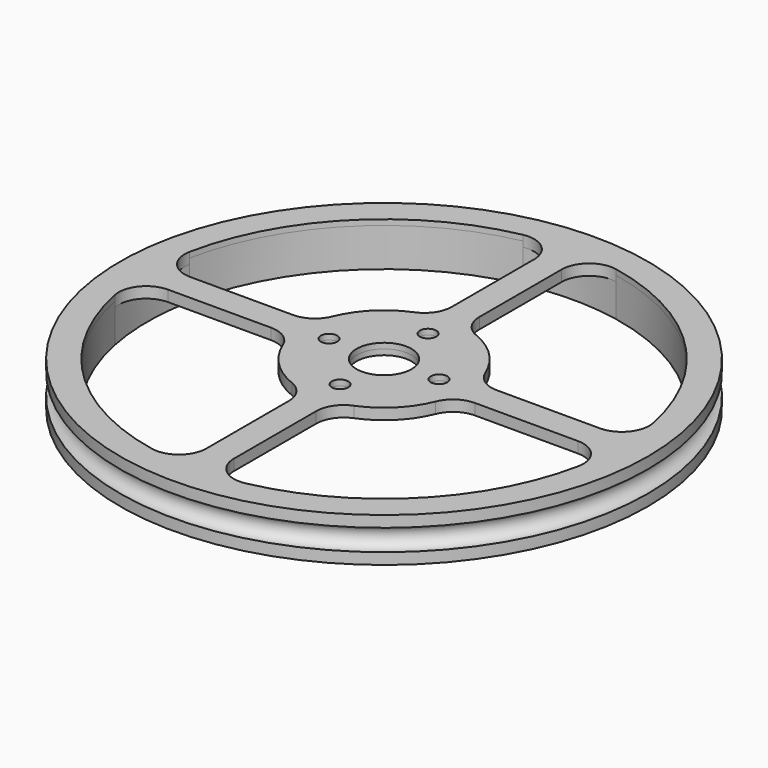
from build123d import *

# Parameters (mm, degrees)
F0_R          = 48
F1_DEPTH      = 1
F1_DEPTH_BACK = 7
F0_R_2        = 1.5
F0_R_3        = 5
F2_DEPTH      = 1
F3_DEPTH      = 1


with BuildPart() as f1:
    # F0 (on Top) → F1 (new body, two sides)
    with BuildSketch(Plane.XY) as f1_sk:
        Circle(F0_R)
        with BuildLine():
            ThreePointArc((8.4868421053, -42.1541636269), (4.2644439289, -42.7880183927), (0, -43))
            ThreePointArc((0, -43), (-4.2644439289, -42.7880183927), (-8.4868421053, -42.1541636269))
            ThreePointArc((-8.4868421053, -42.1541636269), (-30.405591591, -30.405591591), (-42.1541636269, -8.4868421053))
            ThreePointArc((-42.1541636269, -8.4868421053), (-43, 0), (-42.1541636269, 8.4868421053))
            ThreePointArc((-42.1541636269, 8.4868421053), (-30.405591591, 30.405591591), (-8.4868421053, 42.1541636269))
            ThreePointArc((-8.4868421053, 42.1541636269), (0, 43), (8.4868421053, 42.1541636269))
            ThreePointArc((8.4868421053, 42.1541636269), (30.405591591, 30.405591591), (42.1541636269, 8.4868421053))
            ThreePointArc((42.1541636269, 8.4868421053), (42.7880183927, 4.2644439289), (43, 0))
            ThreePointArc((43, 0), (42.7880183927, -4.2644439289), (42.1541636269, -8.4868421053))
            ThreePointArc((42.1541636269, -8.4868421053), (30.405591591, -30.405591591), (8.4868421053, -42.1541636269))
        make_face(mode=Mode.SUBTRACT)
    extrude(amount=F1_DEPTH)
    extrude(f1_sk.sketch, amount=-F1_DEPTH_BACK)



with BuildPart() as f2:
    # F0 (on Top) → F2 (new body, symmetric)
    with BuildSketch(Plane.XY):
        with BuildLine():
            ThreePointArc((0, -15), (2.8652589369, -14.7238001625), (5.625, -13.9053721633))
            ThreePointArc((5.625, -13.9053721633), (10.6066017178, -10.6066017178), (13.9053721633, -5.625))
            ThreePointArc((13.9053721633, -5.625), (14.7238001625, -2.8652589369), (15, 0))
            ThreePointArc((15, 0), (14.7238001625, 2.8652589369), (13.9053721633, 5.625))
            ThreePointArc((13.9053721633, 5.625), (10.6066017178, 10.6066017178), (5.625, 13.9053721633))
            ThreePointArc((5.625, 13.9053721633), (0, 15), (-5.625, 13.9053721633))
            ThreePointArc((-5.625, 13.9053721633), (-10.6066017178, 10.6066017178), (-13.9053721633, 5.625))
            ThreePointArc((-13.9053721633, 5.625), (-15, 0), (-13.9053721633, -5.625))
            ThreePointArc((-13.9053721633, -5.625), (-10.6066017178, -10.6066017178), (-5.625, -13.9053721633))
            ThreePointArc((-5.625, -13.9053721633), (-2.8652589369, -14.7238001625), (0, -15))
        make_face()
        with Locations((0, -10)):
            Circle(F0_R_2, mode=Mode.SUBTRACT)
        with Locations((-10, 0)):
            Circle(F0_R_2, mode=Mode.SUBTRACT)
        Circle(F0_R_3, mode=Mode.SUBTRACT)
        with Locations((10, 0)):
            Circle(F0_R_2, mode=Mode.SUBTRACT)
        with Locations((0, 10)):
            Circle(F0_R_2, mode=Mode.SUBTRACT)
    extrude(amount=F2_DEPTH, both=True)


with BuildPart() as f1_1:
    add(f1.part)

    add(f2.part)  # F3 merges F2
    # F0 (on Top) → F3 (join, symmetric)
    with BuildSketch(Plane.XY):
        with BuildLine():
            Line((0, -43), (0, -15))
            ThreePointArc((0, -15), (-2.8652589369, -14.7238001625), (-5.625, -13.9053721633))
            ThreePointArc((-5.625, -13.9053721633), (-3.3542190121, -15.7454112459), (-2.5, -18.5404962177))
            Line((-2.5, -18.5404962177), (-2.5, -37.2525166935))
            ThreePointArc((-2.5, -37.2525166935), (-4.3325254955, -41.1212510167), (-8.4868421053, -42.1541636269))
            ThreePointArc((-8.4868421053, -42.1541636269), (-4.2644439289, -42.7880183927), (0, -43))
        make_face()
        with BuildLine():
            ThreePointArc((2.5, -18.5404962177), (3.3542190121, -15.7454112459), (5.625, -13.9053721633))
            ThreePointArc((5.625, -13.9053721633), (2.8652589369, -14.7238001625), (0, -15))
            Line((0, -15), (0, -43))
            ThreePointArc((0, -43), (4.2644439289, -42.7880183927), (8.4868421053, -42.1541636269))
            ThreePointArc((8.4868421053, -42.1541636269), (4.3325254955, -41.1212510167), (2.5, -37.2525166935))
            Line((2.5, -37.2525166935), (2.5, -18.5404962177))
        make_face()
        with BuildLine():
            ThreePointArc((15, 0), (14.7238001625, -2.8652589369), (13.9053721633, -5.625))
            ThreePointArc((13.9053721633, -5.625), (15.7454112459, -3.3542190121), (18.5404962177, -2.5))
            Line((18.5404962177, -2.5), (37.2525166935, -2.5))
            ThreePointArc((37.2525166935, -2.5), (41.1212510167, -4.3325254955), (42.1541636269, -8.4868421053))
            ThreePointArc((42.1541636269, -8.4868421053), (42.7880183927, -4.2644439289), (43, 0))
            Line((43, 0), (15, 0))
        make_face()
        with BuildLine():
            ThreePointArc((13.9053721633, 5.625), (14.7238001625, 2.8652589369), (15, 0))
            Line((15, 0), (43, 0))
            ThreePointArc((43, 0), (42.7880183927, 4.2644439289), (42.1541636269, 8.4868421053))
            ThreePointArc((42.1541636269, 8.4868421053), (41.1212510167, 4.3325254955), (37.2525166935, 2.5))
            Line((37.2525166935, 2.5), (18.5404962177, 2.5))
            ThreePointArc((18.5404962177, 2.5), (15.7454112459, 3.3542190121), (13.9053721633, 5.625))
        make_face()
        with BuildLine():
            ThreePointArc((-5.625, 13.9053721633), (0, 15), (5.625, 13.9053721633))
            ThreePointArc((5.625, 13.9053721633), (3.3542190121, 15.7454112459), (2.5, 18.5404962177))
            Line((2.5, 18.5404962177), (2.5, 37.2525166935))
            ThreePointArc((2.5, 37.2525166935), (4.3325254955, 41.1212510167), (8.4868421053, 42.1541636269))
            ThreePointArc((8.4868421053, 42.1541636269), (0, 43), (-8.4868421053, 42.1541636269))
            ThreePointArc((-8.4868421053, 42.1541636269), (-4.3325254955, 41.1212510167), (-2.5, 37.2525166935))
            Line((-2.5, 37.2525166935), (-2.5, 18.5404962177))
            ThreePointArc((-2.5, 18.5404962177), (-3.3542190121, 15.7454112459), (-5.625, 13.9053721633))
        make_face()
        with BuildLine():
            ThreePointArc((-18.5404962177, -2.5), (-15.7454112459, -3.3542190121), (-13.9053721633, -5.625))
            ThreePointArc((-13.9053721633, -5.625), (-15, 0), (-13.9053721633, 5.625))
            ThreePointArc((-13.9053721633, 5.625), (-15.7454112459, 3.3542190121), (-18.5404962177, 2.5))
            Line((-18.5404962177, 2.5), (-37.2525166935, 2.5))
            ThreePointArc((-37.2525166935, 2.5), (-41.1212510167, 4.3325254955), (-42.1541636269, 8.4868421053))
            ThreePointArc((-42.1541636269, 8.4868421053), (-43, 0), (-42.1541636269, -8.4868421053))
            ThreePointArc((-42.1541636269, -8.4868421053), (-41.1212510167, -4.3325254955), (-37.2525166935, -2.5))
            Line((-37.2525166935, -2.5), (-18.5404962177, -2.5))
        make_face()
    extrude(amount=F3_DEPTH, both=True)

    # F4 (on Right) → F5 (revolve, cut)
    with BuildSketch(Plane.YZ):
        with BuildLine():
            Line((48, -4.95), (48, -1.05))
            ThreePointArc((48, -1.05), (46.05, -3), (48, -4.95))
        make_face()
    revolve(axis=Axis((0, 0, -3.6724961751), (0, 0, -1)), mode=Mode.SUBTRACT)


solid = f1_1.part
